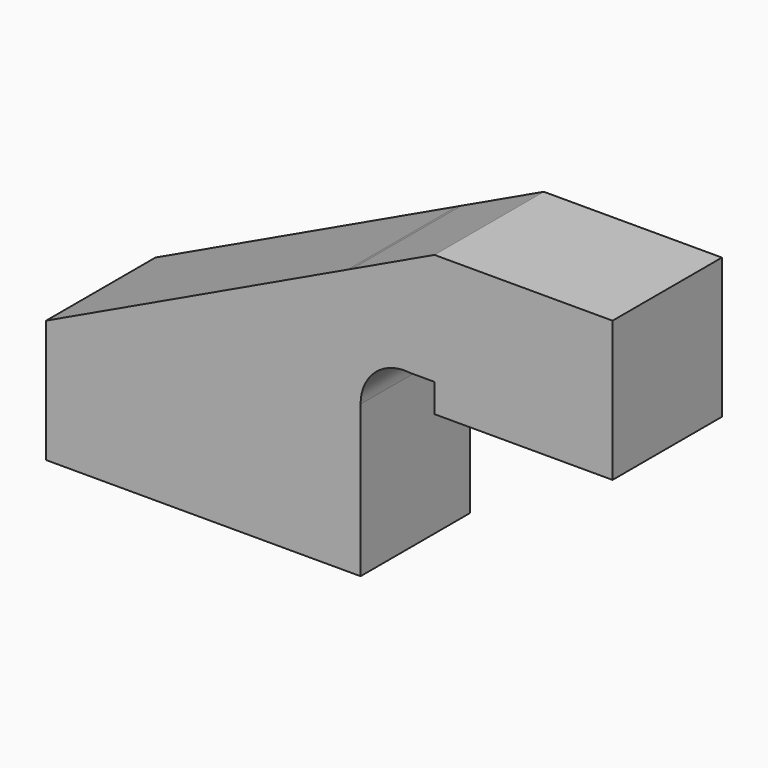
from build123d import *

# Parameters (mm, degrees)
F0_W     = 16.5432430804
F0_H     = 5.2285930142
F0_H_2   = 5.2797589451
F0_H_3   = 15.5384643003
F1_DEPTH = 25.4


with BuildPart() as f1:
    # F0 (on Front) → F1 (new body)
    with BuildSketch(Plane.XZ):
        Polygon((-29.214669019, 11.400138028), (-29.214669019, -11.400138028), (29.214669019, -11.400138028), (29.214669019, 11.400138028), (13.6762047186, 11.400138028), align=None)
        with BuildLine():
            add(Edge.make_bspline(
                [(-29.214669019, 11.400138028), (-10.5295465785, 20.2617670077), (8.155575862, 29.1233959875), (26.8406983024, 37.9850249672)],
                knots=[0, 0, 0, 0, 62.0399904828, 62.0399904828, 62.0399904828, 62.0399904828], degree=3))
            Line((-29.214669019, 11.400138028), (13.6762047186, 11.400138028))
            Line((13.6762047186, 11.400138028), (13.6762047186, 16.7585816234))
            ThreePointArc((13.6762047186, 16.7585816234), (17.2345044889, 29.2472343565), (26.8406983024, 37.9850249672))
        make_face()
        with BuildLine():
            Line((13.6762047186, 11.400138028), (29.214669019, 11.400138028))
            Line((29.214669019, 11.400138028), (29.214669019, 16.7585816234))
            ThreePointArc((29.214669019, 16.7585816234), (31.9669047322, 22.8678129764), (38.3662581444, 24.8542129993))
            Line((38.3662581444, 24.8542129993), (42.9420471191, 24.8542129993))
            Line((42.9420471191, 24.8542129993), (42.9420471191, 40.3926772997))
            Line((42.9420471191, 40.3926772997), (39.0692595726, 40.3926772997))
            ThreePointArc((39.0692595726, 40.3926772997), (33.2055864152, 40.0845606606), (27.5977154023, 38.3440488212))
            add(Edge.make_bspline(
                [(26.8406983024, 37.9850249672), (27.0930373357, 38.1046995852), (27.345376369, 38.2243742032), (27.5977154023, 38.3440488212)],
                knots=[62.0399904828, 62.0399904828, 62.0399904828, 62.0399904828, 62.877828783, 62.877828783, 62.877828783, 62.877828783], degree=3))
            ThreePointArc((26.8406983024, 37.9850249672), (17.2345044889, 29.2472343565), (13.6762047186, 16.7585816234))
            Line((13.6762047186, 16.7585816234), (13.6762047186, 11.400138028))
        make_face()
        with BuildLine():
            ThreePointArc((27.5977154023, 38.3440488212), (27.217619876, 38.1678831015), (26.8406983024, 37.9850249672))
            add(Edge.make_bspline(
                [(26.8406983024, 37.9850249672), (27.0930373357, 38.1046995852), (27.345376369, 38.2243742032), (27.5977154023, 38.3440488212)],
                knots=[62.0399904828, 62.0399904828, 62.0399904828, 62.0399904828, 62.877828783, 62.877828783, 62.877828783, 62.877828783], degree=3))
        make_face()
        with BuildLine():
            add(Edge.make_bspline(
                [(27.5977154023, 38.3440488212), (32.7124926413, 40.7697893188), (37.8272698802, 43.1955298163), (42.9420471191, 45.6212703139)],
                knots=[62.877828783, 62.877828783, 62.877828783, 62.877828783, 79.8603630017, 79.8603630017, 79.8603630017, 79.8603630017], degree=3))
            ThreePointArc((27.5977154023, 38.3440488212), (33.2055864152, 40.0845606606), (39.0692595726, 40.3926772997))
            Line((39.0692595726, 40.3926772997), (42.9420471191, 40.3926772997))
            Line((42.9420471191, 40.3926772997), (42.9420471191, 45.6212703139))
        make_face()
        with Locations((51.2136686593, 43.0069738068)):
            Rectangle(F0_W, F0_H)
        with Locations((51.2136686593, 22.2143335268)):
            Rectangle(F0_W, F0_H_2)
        with Locations((51.2136686593, 32.6234451495)):
            Rectangle(F0_W, F0_H_3)
        Polygon((76.0285332799, 45.6212703139), (59.4852901995, 45.6212703139), (59.4852901995, 40.3926772997), (59.4852901995, 24.8542129993), (59.4852901995, 19.5744540542), (76.0285332799, 19.5744540542), align=None)
    extrude(amount=F1_DEPTH)


solid = f1.part
